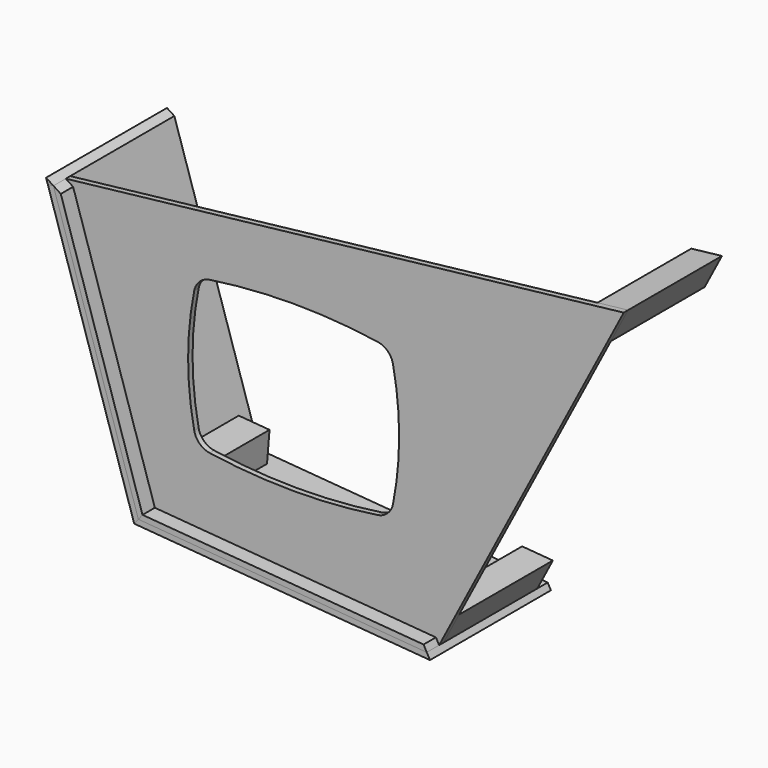
from build123d import *

# Parameters (mm, degrees)
F2_DEPTH      = 9
F4_DEPTH      = 220
F4_DEPTH_BACK = 25
F5_DEPTH      = 220
F5_DEPTH_BACK = 25
F6_DEPTH      = 25
F7_DEPTH      = 25
F10_DEPTH     = 190


with BuildPart() as f2:
    # F1 (on Front) → F2 (new body)
    with BuildSketch(Plane.XZ):
        Polygon((-601.7657060729, 265.5064328389), (-464.0971021196, -165.605785879), (3.4211622742, -203.4229150402), (302.6529489276, 368.4408506737), align=None)
        with BuildLine():
            ThreePointArc((-71.2809765609, 173.3468978927), (-61.3738975589, 73.5150277615), (-71.2809765609, -26.3168423698))
            ThreePointArc((-71.2809765609, -26.3168423698), (-80.0250330385, -42.1627116629), (-96.2921216197, -50.0956762051))
            ThreePointArc((-96.2921216197, -50.0956762051), (-232.4077486992, -60.1403568485), (-368.5233757787, -50.0956762051))
            ThreePointArc((-368.5233757787, -50.0956762051), (-384.7904643599, -42.1627116629), (-393.5345208375, -26.3168423698))
            ThreePointArc((-393.5345208375, -26.3168423698), (-403.4415998395, 73.5150277615), (-393.5345208375, 173.3468978927))
            ThreePointArc((-393.5345208375, 173.3468978927), (-384.7904643599, 189.1927671858), (-368.5233757787, 197.125731728))
            ThreePointArc((-368.5233757787, 197.125731728), (-232.4077486992, 207.1704123714), (-96.2921216197, 197.125731728))
            ThreePointArc((-96.2921216197, 197.125731728), (-80.0250330385, 189.1927671858), (-71.2809765609, 173.3468978927))
        make_face(mode=Mode.SUBTRACT)
    extrude(amount=-F2_DEPTH)


with BuildPart() as f4:
    # F3 (on Front) → F4 (new body, two sides)
    with BuildSketch(Plane.XZ) as f4_sk:
        Polygon((3.4211622742, -203.4229150402), (-464.0971021196, -165.605785879), (-470.8355153758, -174.0901174304), (8.6334902122, -212.8739312278), align=None)
    extrude(amount=-F4_DEPTH)
    extrude(f4_sk.sketch, amount=F4_DEPTH_BACK)


with BuildPart() as f4b:
    # F3 (on Front) → F4, piece 2 (new body, two sides)
    with BuildSketch(Plane.XZ) as f4_2_sk:
        Polygon((-610.8821219424, 264.4688680396), (-601.7657060729, 265.5064328389), (-613.6732371829, 273.2093059424), align=None)
    extrude(amount=-F4_DEPTH)
    extrude(f4_2_sk.sketch, amount=F4_DEPTH_BACK)


with BuildPart() as f5:
    # F3 (on Front) → F5 (new body, two sides)
    with BuildSketch(Plane.XZ) as f5_sk:
        Polygon((-470.8355153758, -174.0901174304), (-464.0971021196, -165.605785879), (-601.7657060729, 265.5064328389), (-610.8821219424, 264.4688680396), align=None)
    extrude(amount=-F5_DEPTH)
    extrude(f5_sk.sketch, amount=F5_DEPTH_BACK)


with BuildPart() as f6:
    # F3 (on Front) → F6 (new body)
    with BuildSketch(Plane.XZ):
        Polygon((-601.7657060729, 265.5064328389), (-464.0971021196, -165.605785879), (-457.3586888634, -157.1214543275), (-589.8581749629, 257.8035597354), align=None)
    extrude(amount=F6_DEPTH)


with BuildPart() as f7:
    # F3 (on Front) → F7 (new body)
    with BuildSketch(Plane.XZ):
        Polygon((-457.3586888634, -157.1214543275), (-464.0971021196, -165.605785879), (3.4211622742, -203.4229150402), (-1.7911656639, -193.9718988526), align=None)
    extrude(amount=F7_DEPTH)


with BuildPart() as f7b:
    # F3 (on Front) → F7, piece 2 (new body)
    with BuildSketch(Plane.XZ):
        Polygon((-470.8355153758, -174.0901174304), (-464.0971021196, -165.605785879), (-601.7657060729, 265.5064328389), (-610.8821219424, 264.4688680396), align=None)
    extrude(amount=F7_DEPTH)


with BuildPart() as f10:
    # F9 (on face) → F10 (new body)
    with BuildSketch(Plane(origin=(0, 9, 0), x_dir=(-1, 0, 0), z_dir=(0, 1, 0))):
        Polygon((-302.6529489276, 368.4408506737), (-274.6537431194, 314.9313908348), (-258.6278079955, 313.1074343152), (-252.9736702823, 362.7867129605), align=None)
    extrude(amount=F10_DEPTH)


with BuildPart() as f10b:
    # F9 (on face) → F10, piece 2 (new body)
    with BuildSketch(Plane(origin=(0, 9, 0), x_dir=(-1, 0, 0), z_dir=(0, 1, 0))):
        Polygon((-28.6036041985, -155.2965905285), (-3.4211622742, -203.4229150402), (25.2649058109, -201.1025249624), (21.2336180232, -151.2653027407), align=None)
    extrude(amount=F10_DEPTH)


with BuildPart() as f10c:
    # F9 (on face) → F10, piece 3 (new body)
    with BuildSketch(Plane(origin=(0, 9, 0), x_dir=(-1, 0, 0), z_dir=(0, 1, 0))):
        Polygon((430.7034560891, -118.1436582337), (434.7347438769, -167.9808804554), (464.0971021196, -165.605785879), (480.5406783108, -114.112370446), align=None)
    extrude(amount=F10_DEPTH)


solid = Compound([f2.part, f4.part, f4b.part, f5.part, f6.part, f7.part, f7b.part, f10.part, f10b.part, f10c.part])
